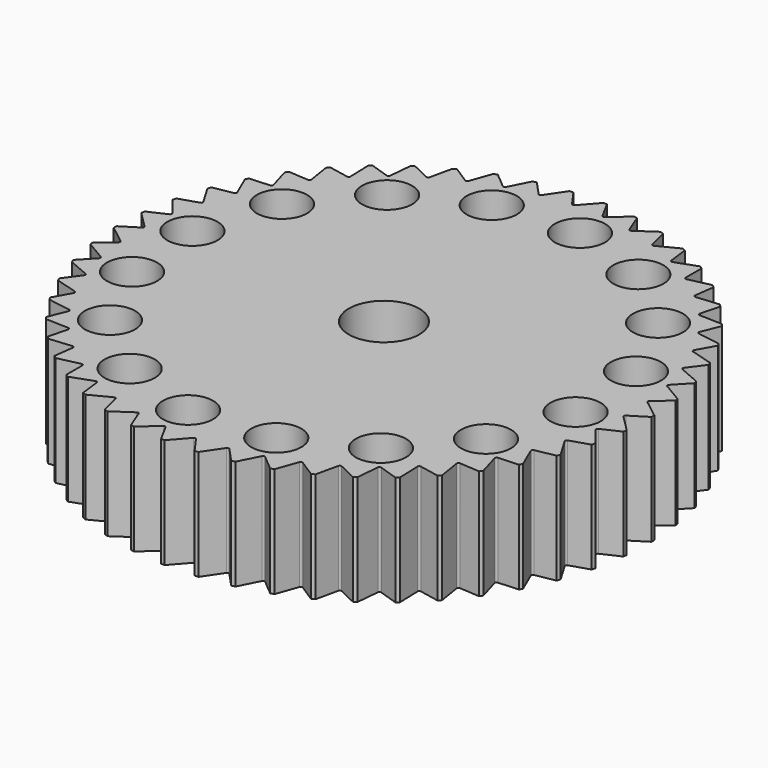
from build123d import *

# Parameters (mm, degrees)
F0_R            = 8
F1_DEPTH        = 25
F2_R            = 5.7035322328
F3_DEPTH        = 25.001
F3_COPIES_COUNT = 16
F5_DEPTH        = 25.001
F5_COPIES_COUNT = 50


# Not quite as in the source:
# - a pattern or mirror of a feature is missing from the dataset's text; its kind, count and spacing are read off the source's solid


with BuildPart() as f1:
    # F0 (on Top) → F1 (new body)
    with BuildSketch(Plane.XY):
        with BuildLine():
            ThreePointArc((1.2819968969, 59.9863024695), (-42.8772656183, -41.9707051775), (60, 0))
            ThreePointArc((60, 0), (45.3667493896, 39.2665003511), (8.6047316725, 59.3797826945))
            Line((8.6047316725, 59.3797826945), (4.3747904217, 52.8191367666))
            Line((4.3747904217, 52.8191367666), (1.2819968969, 59.9863024695))
        make_face()
        with BuildLine():
            ThreePointArc((53, 0), (-38.9927165786, -35.8966301179), (4.3747904217, 52.8191367666))
            ThreePointArc((4.3747904217, 52.8191367666), (38.9927165786, 35.8966301179), (53, 0))
        make_face(mode=Mode.SUBTRACT)
        with BuildLine():
            Line((4.3747904217, 52.8191367666), (8.6047316725, 59.3797826945))
            ThreePointArc((8.6047316725, 59.3797826945), (4.9526575705, 59.7952438158), (1.2819968969, 59.9863024695))
            Line((1.2819968969, 59.9863024695), (4.3747904217, 52.8191367666))
        make_face()
        with BuildLine():
            ThreePointArc((53, 0), (38.9927165786, 35.8966301179), (4.3747904217, 52.8191367666))
            ThreePointArc((4.3747904217, 52.8191367666), (-38.9927165786, -35.8966301179), (53, 0))
        make_face()
        Circle(F0_R, mode=Mode.SUBTRACT)
    extrude(amount=F1_DEPTH)

    # F2 (on face) → F3 (cut, through all)
    with BuildSketch(Plane.XY.offset(25)):
        with Locations((-23.9478349686, -42.3485860229)):
            Circle(F2_R)
    f3 = extrude(amount=-F3_DEPTH, mode=Mode.SUBTRACT)

    # F3_copies: F3 ×16 about axis
    f3_copies_axis = Axis((0, 0, 0), (0, 0, 1))
    for i in range(1, F3_COPIES_COUNT):
        add(f3.rotate(f3_copies_axis, i * 360 / F3_COPIES_COUNT), mode=Mode.SUBTRACT)

    # F4 (on face) → F5 (cut, through all)
    with BuildSketch(Plane.XY.offset(25)):
        with BuildLine():
            ThreePointArc((-56.4392399545, 20.3620282232), (-57.4908112019, 17.1699338189), (-58.362000737, 13.9239674654))
            Line((-58.362000737, 13.9239674654), (-54.0138308591, 15.3096202723))
            ThreePointArc((-54.0138308591, 15.3096202723), (-53.7614352022, 15.5484764635), (-53.7911914471, 15.8946995326))
            Line((-53.7911914471, 15.8946995326), (-56.4392399545, 20.3620282232))
        make_face()
    f5 = extrude(amount=-F5_DEPTH, mode=Mode.SUBTRACT)

    # F5_copies: F5 ×50 about axis
    f5_copies_axis = Axis((0, 0, 0), (0, 0, 1))
    for i in range(1, F5_COPIES_COUNT):
        add(f5.rotate(f5_copies_axis, i * 360 / F5_COPIES_COUNT), mode=Mode.SUBTRACT)


solid = f1.part
